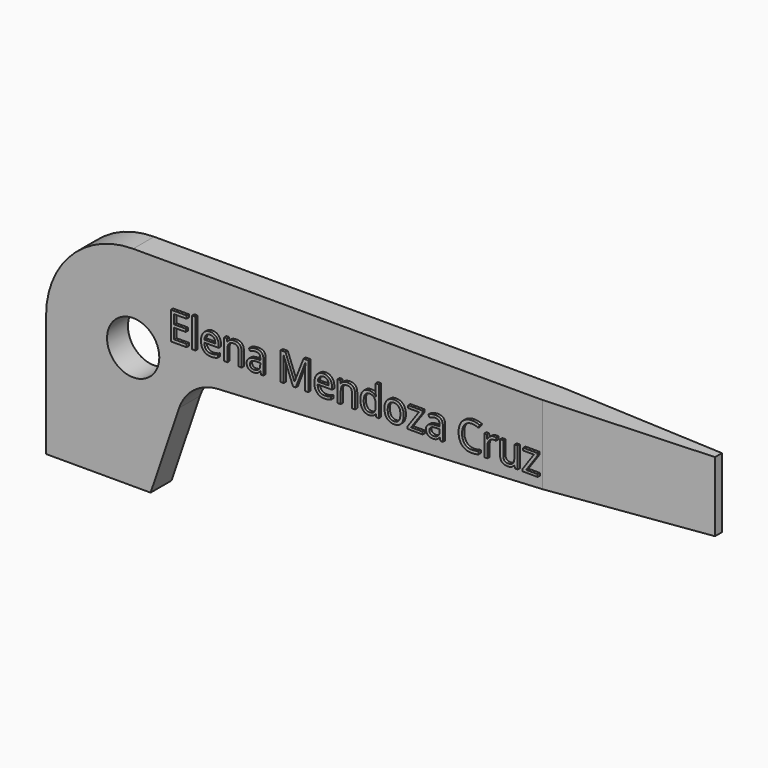
from build123d import *

# Parameters (mm, degrees)
F1_DEPTH     = 2.38125
F2_R         = 2.38125
F3_DEPTH     = 25.4
F5_DEPTH     = 25.4
F6_TEXT_SIZE = 3.5711551813
F7_DEPTH     = 0.254


# Not quite as in the source:
# - Text() gives the source's letters only with a copy of the font that has no kerning and outlines rounded to 1/6400 em; it was checked with that copy


with BuildPart() as f1:
    # F0 (on Front) → F1 (new body)
    with BuildSketch(Plane.XZ):
        with BuildLine():
            Line((60.325, 19.05), (7.9375, 19.05))
            ThreePointArc((7.9375, 19.05), (2.3248399243, 16.7251600757), (0, 11.1125))
            Line((0, 11.1125), (0, 0))
            Line((0, 0), (9.525, 0))
            Line((9.525, 0), (12.1173647876, 7.6271664624))
            ThreePointArc((12.1173647876, 7.6271664624), (13.4786145605, 9.5135918491), (15.6631963617, 10.3130942181))
            Line((15.6631963617, 10.3130942181), (60.325, 12.7))
            Line((60.325, 12.7), (60.325, 19.05))
        make_face()
    extrude(amount=F1_DEPTH)

    # F2 (on face) → F3 (cut)
    with BuildSketch(Plane.XZ.offset(2.38125)):
        with Locations((7.9375, 11.1125)):
            Circle(F2_R)
    extrude(amount=-F3_DEPTH, mode=Mode.SUBTRACT)

    # F4 (on face) → F5 (cut)
    with BuildSketch(Plane.XY.offset(19.05)):
        Polygon((60.325, -2.38125), (60.325, -1.5875), (45.24375, -2.38125), align=None)
        Polygon((60.325, 0), (45.24375, 0), (60.325, -0.79375), align=None)
    extrude(amount=-F5_DEPTH, mode=Mode.SUBTRACT)

    # F6 (on face) → F7 (join)
    with BuildSketch(Plane.XZ.offset(2.38125)):
        with Locations((11.2312868632, 12.9007670482)):
            Text('Elena Mendoza Cruz', F6_TEXT_SIZE, font='Open Sans', text_align=(TextAlign.LEFT, TextAlign.BOTTOM))
    extrude(amount=F7_DEPTH)


solid = f1.part
